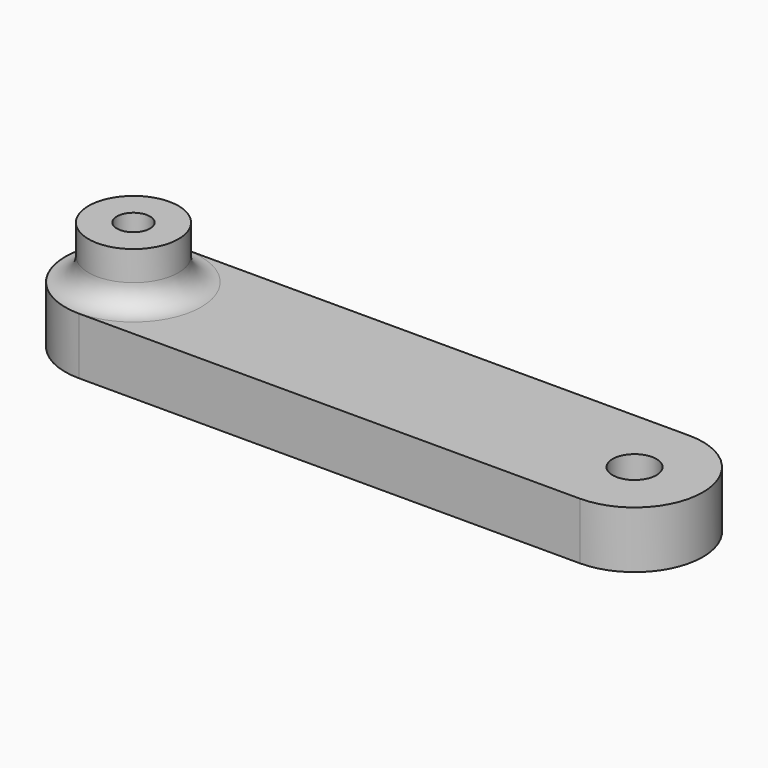
from build123d import *

# Parameters (mm, degrees)
F0_R          = 1.925
F1_DEPTH      = 5
F2_R          = 3.95
F2_R_2        = 1.45
F3_DEPTH      = 4.6
F3_DEPTH_BACK = 5
F4_R          = 2


with BuildPart() as f1:
    # F0 (on Top) → F1 (new body)
    with BuildSketch(Plane.XY):
        with BuildLine():
            Line((-44, -6), (0, -6))
            ThreePointArc((0, -6), (6, 0), (0, 6))
            Line((0, 6), (-44, 6))
            ThreePointArc((-44, 6), (-50, 0), (-44, -6))
        make_face()
        with Locations((-44, 0)):
            Circle(F0_R, mode=Mode.SUBTRACT)
        Circle(F0_R, mode=Mode.SUBTRACT)
    extrude(amount=F1_DEPTH)

    # F2 (on face) → F3 (join, two sides)
    with BuildSketch(Plane.XY.offset(5)) as f3_sk:
        with Locations((-44, 0)):
            Circle(F2_R)
        with Locations((-44, 0)):
            Circle(F2_R_2, mode=Mode.SUBTRACT)
    extrude(amount=F3_DEPTH)
    extrude(f3_sk.sketch, amount=-F3_DEPTH_BACK)

    # F4
    f4_edges = [f1.edges().sort_by_distance(p)[0] for p in [
        (-47.95, 0, 5),
    ]]
    fillet(f4_edges, radius=F4_R)


solid = f1.part
